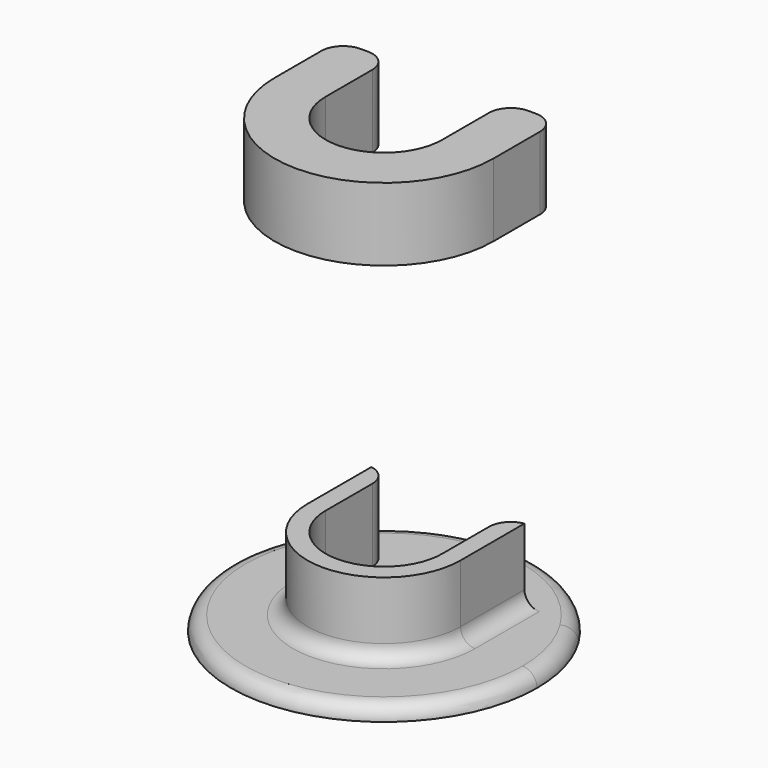
from build123d import *

# Parameters (mm, degrees)
F1_DEPTH = 2
F2_DEPTH = 10
F3_R     = 1.99999
F4_R     = 3
F7_DEPTH = 10
F8_R     = 3


# Not quite as in the source:
# - a fillet or chamfer is up to 0.001 mm smaller than in the source, because OpenCascade refuses the exact size


with BuildPart() as f1:
    # F0 (on Top) → F1 (new body)
    with BuildSketch(Plane.XY):
        with BuildLine():
            ThreePointArc((-17.88854382, 11), (-5.7157930237, -20.2071697699), (21, 0))
            ThreePointArc((21, 0), (20.2071697699, 5.7157930237), (17.88854382, 11))
            Line((17.88854382, 11), (10.5, 11))
            Line((10.5, 11), (10.5, 0))
            ThreePointArc((10.5, 0), (0, -10.5), (-10.5, 0))
            Line((-10.5, 0), (-10.5, 11))
            Line((-10.5, 11), (-17.88854382, 11))
        make_face()
        with BuildLine():
            Line((10.5, 11), (17.88854382, 11))
            ThreePointArc((17.88854382, 11), (0, 21), (-17.88854382, 11))
            Line((-17.88854382, 11), (-10.5, 11))
            Line((-10.5, 11), (-8, 11))
            Line((-8, 11), (8, 11))
            Line((8, 11), (10.5, 11))
        make_face()
        with BuildLine():
            ThreePointArc((-8, 0), (0, -8), (8, 0))
            ThreePointArc((8, 0), (0, 8), (-8, 0))
        make_face()
        with BuildLine():
            Line((8, 0), (8, 6.8007352544))
            ThreePointArc((8, 6.8007352544), (0, 10.5), (-8, 6.8007352544))
            Line((-8, 6.8007352544), (-8, 0))
            ThreePointArc((-8, 0), (0, 8), (8, 0))
        make_face()
        with BuildLine():
            ThreePointArc((-10.5, 0), (0, -10.5), (10.5, 0))
            ThreePointArc((10.5, 0), (9.8552016722, 3.6228441865), (8, 6.8007352544))
            Line((8, 6.8007352544), (8, 0))
            ThreePointArc((8, 0), (0, -8), (-8, 0))
            Line((-8, 0), (-8, 6.8007352544))
            ThreePointArc((-8, 6.8007352544), (-9.8552016722, 3.6228441865), (-10.5, 0))
        make_face()
        with BuildLine():
            Line((-8, 11), (-10.5, 11))
            Line((-10.5, 11), (-10.5, 0))
            ThreePointArc((-10.5, 0), (-9.8552016722, 3.6228441865), (-8, 6.8007352544))
            Line((-8, 6.8007352544), (-8, 11))
        make_face()
        with BuildLine():
            Line((8, 6.8007352544), (8, 11))
            Line((8, 11), (-8, 11))
            Line((-8, 11), (-8, 6.8007352544))
            ThreePointArc((-8, 6.8007352544), (0, 10.5), (8, 6.8007352544))
        make_face()
        with BuildLine():
            Line((10.5, 0), (10.5, 11))
            Line((10.5, 11), (8, 11))
            Line((8, 11), (8, 6.8007352544))
            ThreePointArc((8, 6.8007352544), (9.8552016722, 3.6228441865), (10.5, 0))
        make_face()
    extrude(amount=-F1_DEPTH)

    # F0 (on Top) → F2 (join)
    with BuildSketch(Plane.XY):
        with BuildLine():
            Line((10.5, 0), (10.5, 11))
            Line((10.5, 11), (8, 11))
            Line((8, 11), (8, 6.8007352544))
            ThreePointArc((8, 6.8007352544), (9.8552016722, 3.6228441865), (10.5, 0))
        make_face()
        with BuildLine():
            ThreePointArc((-10.5, 0), (0, -10.5), (10.5, 0))
            ThreePointArc((10.5, 0), (9.8552016722, 3.6228441865), (8, 6.8007352544))
            Line((8, 6.8007352544), (8, 0))
            ThreePointArc((8, 0), (0, -8), (-8, 0))
            Line((-8, 0), (-8, 6.8007352544))
            ThreePointArc((-8, 6.8007352544), (-9.8552016722, 3.6228441865), (-10.5, 0))
        make_face()
        with BuildLine():
            Line((-8, 11), (-10.5, 11))
            Line((-10.5, 11), (-10.5, 0))
            ThreePointArc((-10.5, 0), (-9.8552016722, 3.6228441865), (-8, 6.8007352544))
            Line((-8, 6.8007352544), (-8, 11))
        make_face()
    extrude(amount=F2_DEPTH)

    # F3 (radius 2 in the source; OpenCascade refuses exactly that, so slightly less here)
    f3_edges = [f1.edges().sort_by_distance(p)[0] for p in [
        (-21, 0, 0),
        (0, -10.5, 0),
        (10.5, 5.5, 0),
        (-10.5, 5.5, 0),
    ]]
    fillet(f3_edges, radius=F3_R)

    # F4
    f4_edges = [f1.edges().sort_by_distance(p)[0] for p in [
        (-8, 11, 5),
        (8, 11, 5),
    ]]
    fillet(f4_edges, radius=F4_R)


with BuildPart() as f7:
    # F6 (on offset) → F7 (new body)
    with BuildSketch(Plane.XY.offset(50)):
        with BuildLine():
            Line((-15, 11), (-15, 0))
            ThreePointArc((-15, 0), (-13.7471921753, 6.0012254829), (-10.1980390272, 11))
            Line((-10.1980390272, 11), (-15, 11))
        make_face()
        with BuildLine():
            ThreePointArc((-10.1980390272, 11), (-13.7471921753, 6.0012254829), (-15, 0))
            ThreePointArc((-15, 0), (0, -15), (15, 0))
            ThreePointArc((15, 0), (13.7471921753, 6.0012254829), (10.1980390272, 11))
            Line((10.1980390272, 11), (8, 11))
            Line((8, 11), (8, 0))
            ThreePointArc((8, 0), (0, -8), (-8, 0))
            Line((-8, 0), (-8, 11))
            Line((-8, 11), (-10.1980390272, 11))
        make_face()
        with BuildLine():
            ThreePointArc((10.1980390272, 11), (13.7471921753, 6.0012254829), (15, 0))
            Line((15, 0), (15, 11))
            Line((15, 11), (10.1980390272, 11))
        make_face()
    extrude(amount=F7_DEPTH)

    # F8
    f8_edges = [f7.edges().sort_by_distance(p)[0] for p in [
        (-8, 11, 55),
        (8, 11, 55),
        (-15, 11, 55),
        (15, 11, 55),
    ]]
    fillet(f8_edges, radius=F8_R)


solid = Compound([f1.part, f7.part])
